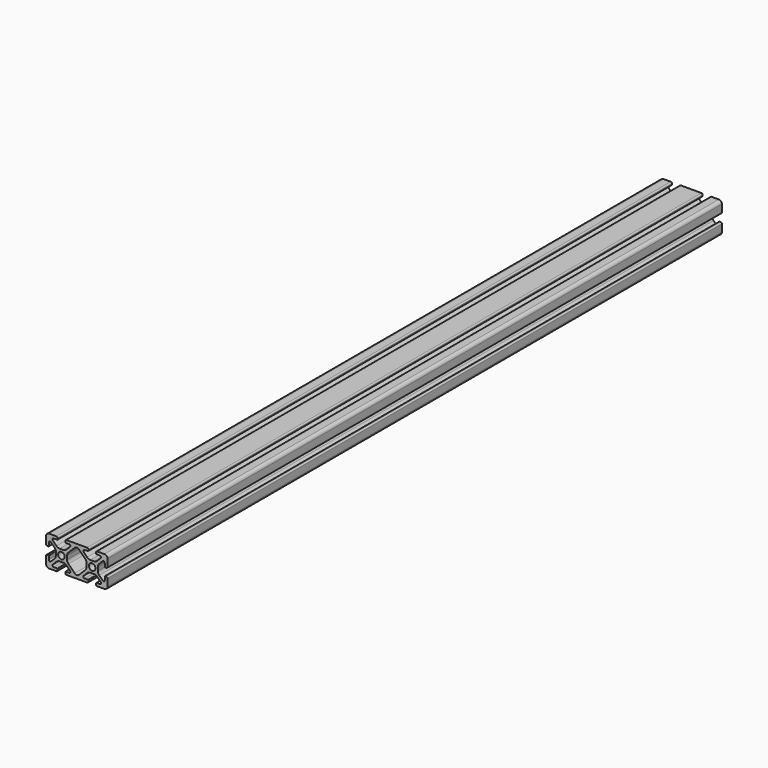
from build123d import *

# Parameters (mm, degrees)
F0_R     = 2.15
F1_DEPTH = 250


# Not quite as in the source:
# - ends of sketch curves that miss each other by under 0.0002 mm in the source are joined


with BuildPart() as f1:
    # F0 (on Front) → F1 (new body, symmetric)
    with BuildSketch(Plane.XZ):
        with BuildLine():
            Line((7.5, 8.5), (7.5, 9.2))
            ThreePointArc((7.5, 9.2), (7.2656854249, 9.7656854249), (6.7, 10))
            Line((6.7, 10), (-6.7, 10))
            ThreePointArc((-6.7, 10), (-7.2656854249, 9.7656854249), (-7.5, 9.2))
            Line((-7.5, 9.2), (-7.5, 8.5))
            ThreePointArc((-7.5, 8.5), (-7.4121320344, 8.2878679656), (-7.2, 8.2))
            Line((-7.2, 8.2), (-5.004162, 8.2))
            ThreePointArc((-5.004162, 8.2), (-4.2650582387, 7.7061464193), (-4.4384770751, 6.8343140751))
            Line((-4.4384770751, 6.8343140751), (-6.744114, 4.528679))
            ThreePointArc((-6.744114, 4.528679), (-7.7173840295, 3.8783612672), (-8.865434, 3.65))
            Line((-8.865434, 3.65), (-11.134566, 3.65))
            ThreePointArc((-11.134566, 3.65), (-12.2826159705, 3.8783612672), (-13.2558858436, 4.5286791564))
            Line((-13.2558858436, 4.5286791564), (-15.561523, 6.834314))
            ThreePointArc((-15.561523, 6.834314), (-15.7349417613, 7.7061464193), (-14.995838, 8.2))
            Line((-14.995838, 8.2), (-12.8, 8.2))
            ThreePointArc((-12.8, 8.2), (-12.5878679656, 8.2878679656), (-12.5, 8.5))
            Line((-12.5, 8.5), (-12.5, 9.2))
            ThreePointArc((-12.5, 9.2), (-12.7343145751, 9.7656854249), (-13.3, 10))
            Line((-13.3, 10), (-18, 10))
            ThreePointArc((-18, 10), (-19.4142135624, 9.4142135624), (-20, 8))
            Line((-20, 8), (-20, 3.3))
            ThreePointArc((-20, 3.3), (-19.7656854249, 2.7343145751), (-19.2, 2.5))
            Line((-19.2, 2.5), (-18.500003, 2.5))
            ThreePointArc((-18.500003, 2.5), (-18.2878709656, 2.5878679656), (-18.200003, 2.8))
            Line((-18.200003, 2.8), (-18.200003, 4.995834))
            ThreePointArc((-18.200003, 4.995834), (-17.7061497459, 5.734937626), (-16.8343175751, 5.5615194249))
            Line((-16.8343175751, 5.5615194249), (-14.528682, 3.255884))
            ThreePointArc((-14.528682, 3.255884), (-13.8783635378, 2.2826136237), (-13.650002, 1.134563))
            Line((-13.650002, 1.134563), (-13.650002, -1.134563))
            ThreePointArc((-13.650002, -1.134563), (-13.8783635378, -2.2826136237), (-14.5286821564, -3.2558838436))
            Line((-14.5286821564, -3.2558838436), (-16.834318, -5.561519))
            ThreePointArc((-16.834318, -5.561519), (-17.7061497459, -5.734937626), (-18.200003, -4.995834))
            Line((-18.200003, -4.995834), (-18.200003, -2.8))
            ThreePointArc((-18.200003, -2.8), (-18.2878709656, -2.5878679656), (-18.500003, -2.5))
            Line((-18.500003, -2.5), (-19.2, -2.5))
            ThreePointArc((-19.2, -2.5), (-19.7656854249, -2.7343145751), (-20, -3.3))
            Line((-20, -3.3), (-20, -8))
            ThreePointArc((-20, -8), (-19.4142135624, -9.4142135624), (-18, -10))
            Line((-18, -10), (-13.3, -10))
            ThreePointArc((-13.3, -10), (-12.7343145751, -9.7656854249), (-12.5, -9.2))
            Line((-12.5, -9.2), (-12.5, -8.5))
            ThreePointArc((-12.5, -8.5), (-12.5878679656, -8.2878679656), (-12.8, -8.2))
            Line((-12.8, -8.2), (-14.995838, -8.2))
            ThreePointArc((-14.995838, -8.2), (-15.7349417613, -7.7061464193), (-15.5615229249, -6.8343140751))
            Line((-15.5615229249, -6.8343140751), (-13.255886, -4.528679))
            ThreePointArc((-13.255886, -4.528679), (-12.2826159705, -3.8783612672), (-11.134566, -3.65))
            Line((-11.134566, -3.65), (-8.865434, -3.65))
            ThreePointArc((-8.865434, -3.65), (-7.7173840295, -3.8783612672), (-6.7441141564, -4.5286791564))
            Line((-6.7441141564, -4.5286791564), (-4.438477, -6.834314))
            ThreePointArc((-4.438477, -6.834314), (-4.2650582387, -7.7061464193), (-5.004162, -8.2))
            Line((-5.004162, -8.2), (-7.2, -8.2))
            ThreePointArc((-7.2, -8.2), (-7.4121320344, -8.2878679656), (-7.5, -8.5))
            Line((-7.5, -8.5), (-7.5, -9.2))
            ThreePointArc((-7.5, -9.2), (-7.2656854249, -9.7656854249), (-6.7, -10))
            Line((-6.7, -10), (6.7, -10))
            ThreePointArc((6.7, -10), (7.2656854249, -9.7656854249), (7.5, -9.2))
            Line((7.5, -9.2), (7.5, -8.5))
            ThreePointArc((7.5, -8.5), (7.4121320344, -8.2878679656), (7.2, -8.2))
            Line((7.2, -8.2), (5.004162, -8.2))
            ThreePointArc((5.004162, -8.2), (4.2650582387, -7.7061464193), (4.4384770751, -6.8343140751))
            Line((4.4384770751, -6.8343140751), (6.744114, -4.528679))
            ThreePointArc((6.744114, -4.528679), (7.7173840295, -3.8783612672), (8.865434, -3.65))
            Line((8.865434, -3.65), (11.134566, -3.65))
            ThreePointArc((11.134566, -3.65), (12.2826159705, -3.8783612672), (13.2558858436, -4.5286791564))
            Line((13.2558858436, -4.5286791564), (15.561523, -6.834314))
            ThreePointArc((15.561523, -6.834314), (15.7349417613, -7.7061464193), (14.995838, -8.2))
            Line((14.995838, -8.2), (12.8, -8.2))
            ThreePointArc((12.8, -8.2), (12.5878679656, -8.2878679656), (12.5, -8.5))
            Line((12.5, -8.5), (12.5, -9.2))
            ThreePointArc((12.5, -9.2), (12.7343145751, -9.7656854249), (13.3, -10))
            Line((13.3, -10), (18, -10))
            ThreePointArc((18, -10), (19.4142135624, -9.4142135624), (20, -8))
            Line((20, -8), (20, -3.3))
            ThreePointArc((20, -3.3), (19.7656854249, -2.7343145751), (19.2, -2.5))
            Line((19.2, -2.5), (18.500003, -2.5))
            ThreePointArc((18.500003, -2.5), (18.2878709656, -2.5878679656), (18.200003, -2.8))
            Line((18.200003, -2.8), (18.200003, -4.995834))
            ThreePointArc((18.200003, -4.995834), (17.7061497459, -5.734937626), (16.8343175751, -5.5615194249))
            Line((16.8343175751, -5.5615194249), (14.528682, -3.255884))
            ThreePointArc((14.528682, -3.255884), (13.8783635378, -2.2826136237), (13.650002, -1.134563))
            Line((13.650002, -1.134563), (13.650002, 1.134563))
            ThreePointArc((13.650002, 1.134563), (13.8783635378, 2.2826136237), (14.5286821564, 3.2558838436))
            Line((14.5286821564, 3.2558838436), (16.834318, 5.561519))
            ThreePointArc((16.834318, 5.561519), (17.7061497459, 5.734937626), (18.200003, 4.995834))
            Line((18.200003, 4.995834), (18.200003, 2.8))
            ThreePointArc((18.200003, 2.8), (18.2878709656, 2.5878679656), (18.500003, 2.5))
            Line((18.500003, 2.5), (19.2, 2.5))
            ThreePointArc((19.2, 2.5), (19.7656854249, 2.7343145751), (20, 3.3))
            Line((20, 3.3), (20, 8))
            ThreePointArc((20, 8), (19.4142135624, 9.4142135624), (18, 10))
            Line((18, 10), (13.3, 10))
            ThreePointArc((13.3, 10), (12.7343145751, 9.7656854249), (12.5, 9.2))
            Line((12.5, 9.2), (12.5, 8.5))
            ThreePointArc((12.5, 8.5), (12.5878679656, 8.2878679656), (12.8, 8.2))
            Line((12.8, 8.2), (14.995838, 8.2))
            ThreePointArc((14.995838, 8.2), (15.7349417613, 7.7061464193), (15.5615229249, 6.8343140751))
            Line((15.5615229249, 6.8343140751), (13.255886, 4.528679))
            ThreePointArc((13.255886, 4.528679), (12.2826159705, 3.8783612672), (11.134566, 3.65))
            Line((11.134566, 3.65), (8.865434, 3.65))
            ThreePointArc((8.865434, 3.65), (7.7173840295, 3.8783612672), (6.7441141564, 4.5286791564))
            Line((6.7441141564, 4.5286791564), (4.438477, 6.834314))
            ThreePointArc((4.438477, 6.834314), (4.2650582387, 7.7061464193), (5.004162, 8.2))
            Line((5.004162, 8.2), (7.2, 8.2))
            ThreePointArc((7.2, 8.2), (7.4121320344, 8.2878679656), (7.5, 8.5))
        make_face()
        with Locations((-10, 0)):
            Circle(F0_R, mode=Mode.SUBTRACT)
        with BuildLine():
            ThreePointArc((-1.4142130624, 7.3129870624), (0, 7.898773), (1.4142130624, 7.3129870624))
            Line((1.4142130624, 7.3129870624), (5.471318, 3.255884))
            ThreePointArc((5.471318, 3.255884), (6.1216364622, 2.2826136237), (6.349998, 1.134563))
            Line((6.349998, 1.134563), (6.349998, -1.134563))
            ThreePointArc((6.349998, -1.134563), (6.1216364622, -2.2826136237), (5.4713178436, -3.2558838436))
            Line((5.4713178436, -3.2558838436), (1.414213, -7.312987))
            ThreePointArc((1.414213, -7.312987), (0, -7.898773), (-1.4142130624, -7.3129870624))
            Line((-1.4142130624, -7.3129870624), (-5.471318, -3.255884))
            ThreePointArc((-5.471318, -3.255884), (-6.1216364622, -2.2826136237), (-6.349998, -1.134563))
            Line((-6.349998, -1.134563), (-6.349998, 1.134563))
            ThreePointArc((-6.349998, 1.134563), (-6.1216364622, 2.2826136237), (-5.4713178436, 3.2558838436))
            Line((-5.4713178436, 3.2558838436), (-1.4142130624, 7.3129870624))
        make_face(mode=Mode.SUBTRACT)
        with Locations((10, 0)):
            Circle(F0_R, mode=Mode.SUBTRACT)
    extrude(amount=F1_DEPTH, both=True)


solid = f1.part
